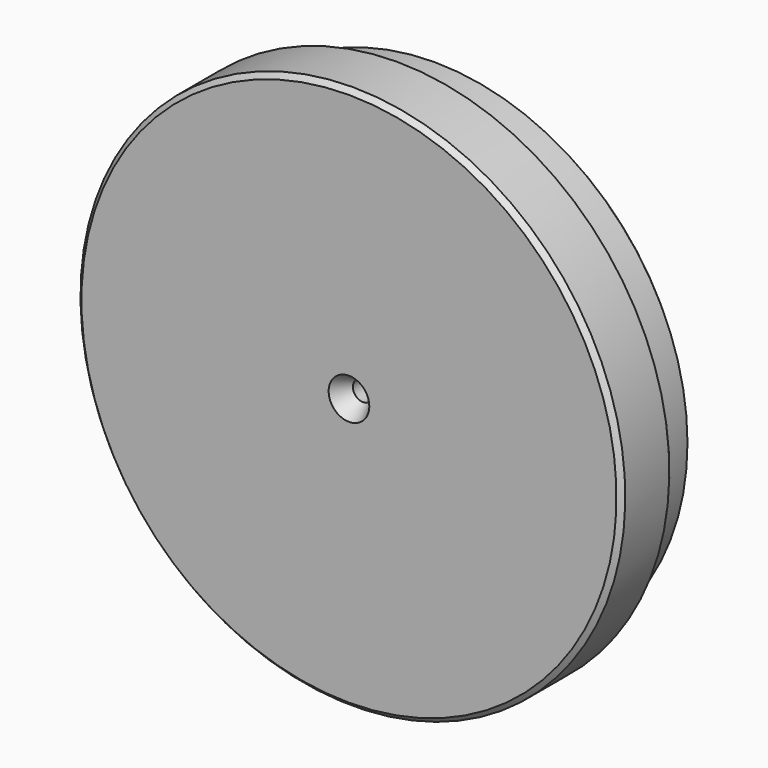
from build123d import *

# Parameters (mm, degrees)
F2_R    = 0.508
F3_SIZE = 1.524


with BuildPart() as f1:
    # F0 (on Right) → F1 (revolve)
    with BuildSketch(Plane.YZ):
        Polygon((-21.1680062206, 0), (0, 0), (0, 79.00924), (-14.6116351058, 79.00924), (-15.3736351058, 78.24724), (-15.875, 78.24724), (-15.875, 79.00924), (-15.875, 85.09), (-34.925, 85.09), (-34.925, 6.35), (-29.425738686, 3.175), (-23.075738686, 3.175), align=None)
    revolve(axis=Axis((0, -21.1680062206, 0), (0, 1, 0)))

    # F2
    f2_edges = [f1.edges().sort_by_distance(p)[0] for p in [
        (0, -15.875, -85.09),
    ]]
    fillet(f2_edges, radius=F2_R)

    # F3
    f3_edges = [f1.edges().sort_by_distance(p)[0] for p in [
        (0, 0, -79.00924),
        (0, -34.925, -85.09),
    ]]
    chamfer(f3_edges, length=F3_SIZE)


solid = f1.part
